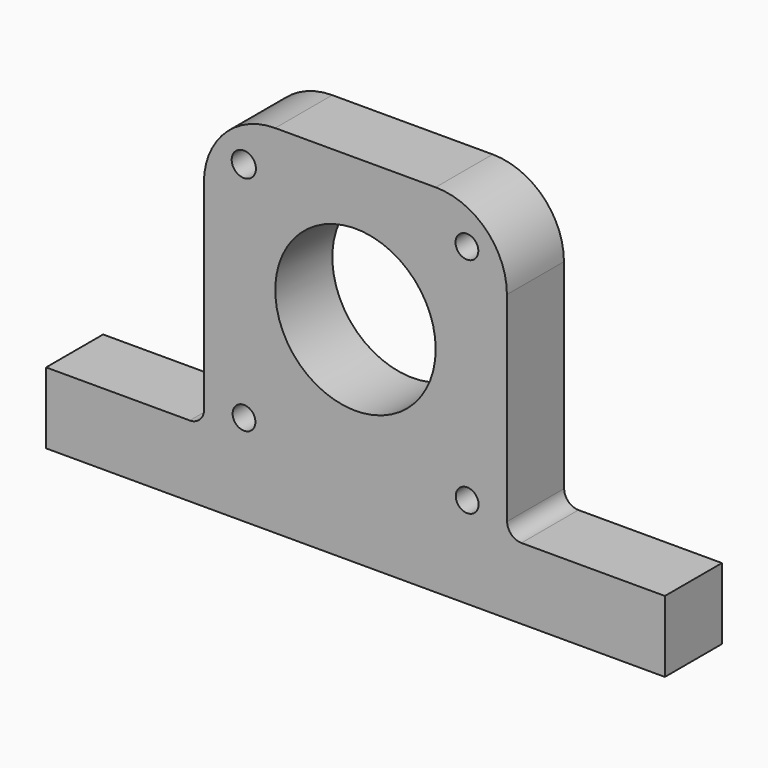
from build123d import *

# Parameters (mm, degrees)
F0_R     = 1.6
F0_R_2   = 1.7
F0_R_3   = 11.25
F1_DEPTH = 10
F2_R     = 2


# Not quite as in the source:
# - a feature of the source that left no trace in its solid (it failed there, or was rolled back) is left out


with BuildPart() as f1:
    # F0 (on Front) → F1 (new body)
    with BuildSketch(Plane.XZ):
        with BuildLine():
            Line((11.2397133785, 19.9999894063), (-11.2602985395, 19.9999894063))
            ThreePointArc((-11.2602985395, 19.9999894063), (-18.3350043941, 17.0674173026), (-21.2602932426, 9.9896968203))
            Line((-21.2602932426, 9.9896968203), (-21.229426084, -19.9999894063))
            Line((-21.229426084, -19.9999894063), (-43.3949531186, -19.9999894063))
            Line((-43.3949531186, -19.9999894063), (-43.3949531186, -29.9999894063))
            Line((-43.3949531186, -29.9999894063), (43.3949531186, -29.9999894063))
            Line((43.3949531186, -29.9999894063), (43.3949531186, -19.9999894063))
            Line((43.3949531186, -19.9999894063), (21.2705964277, -19.9999894063))
            Line((21.2705964277, -19.9999894063), (21.2397080816, 10.0102819922))
            ThreePointArc((21.2397080816, 10.0102819922), (18.3071412749, 17.0746952609), (11.2397133785, 19.9999894063))
        make_face()
        with Locations((-15.6323080096, -17.1999894063)):
            Circle(F0_R, mode=Mode.SUBTRACT)
        with Locations((15.6677115429, -17.1999961863)):
            Circle(F0_R, mode=Mode.SUBTRACT)
        with Locations((-15.6645237988, 14.0999894063)):
            Circle(F0_R_2, mode=Mode.SUBTRACT)
        Circle(F0_R_3, mode=Mode.SUBTRACT)
        with Locations((15.629426084, 14.0999894063)):
            Circle(F0_R, mode=Mode.SUBTRACT)
    extrude(amount=F1_DEPTH)

    # F2
    f2_edges = [f1.edges().sort_by_distance(p)[0] for p in [
        (21.270596, -5, -19.999989),
        (-21.229426, -5, -19.999989),
    ]]
    fillet(f2_edges, radius=F2_R)


solid = f1.part
